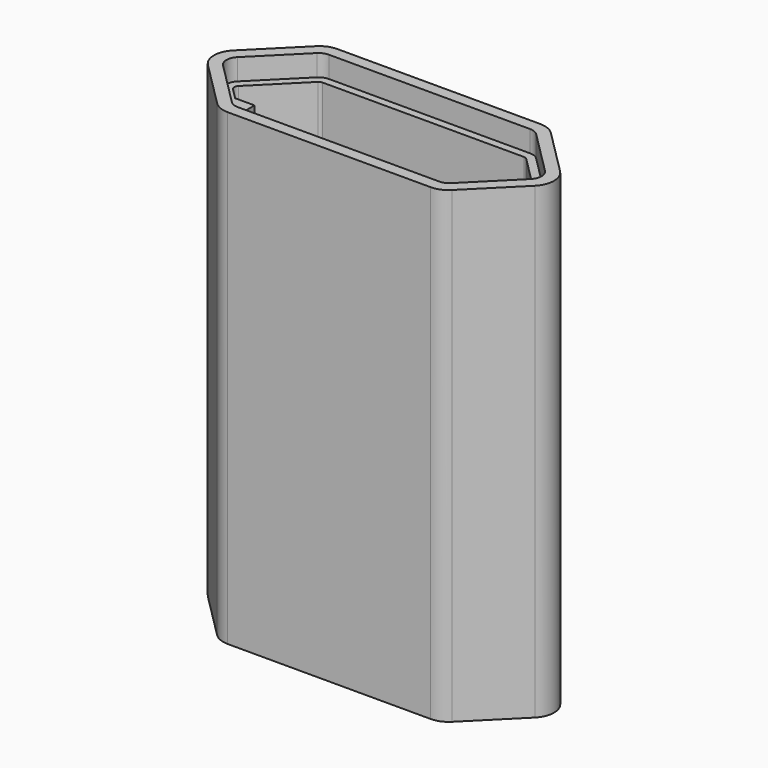
from build123d import *

# Parameters (mm, degrees)
F1_DEPTH     = 2
F2_DEPTH     = 5
F3_DEPTH     = 44
F4_DEPTH     = 46.2
F6_T1_DEPTH  = 6.8
F6_T3_DEPTH  = 13.8
F6_T9_DEPTH  = 16.371682988
F6_T15_DEPTH = 9.371682988
F6_T24_DEPTH = 9.371682988
F6_T30_DEPTH = 16.371682988
F6_T39_DEPTH = 16.371682988
F6_T45_DEPTH = 9.371682988
F6_T54_DEPTH = 16.371682988
F6_T60_DEPTH = 9.371682988


# Not quite as in the source:
# - a fillet or chamfer that OpenCascade refuses, or shapes differently, is made with other operations: its cross-section is extruded or revolved along the edge and cut away or added
# - a feature names something its author has since deleted; it is built from what else it names


with BuildPart() as f1:
    # F0 (on Top) → F1 (new body)
    with BuildSketch(Plane.XY):
        with BuildLine():
            Line((10.3671572875, 5.05), (0, 5.05))
            Line((0, 5.05), (0, 4.2))
            Line((0, 4.2), (7.7, 4.2))
            Line((7.7, 4.2), (7.7, -4.2))
            Line((7.7, -4.2), (0, -4.2))
            Line((0, -4.2), (0, -5.05))
            Line((0, -5.05), (10.3671572875, -5.05))
            ThreePointArc((10.3671572875, -5.05), (10.5584990037, -5.0119397663), (10.7207106781, -4.9035533906))
            Line((10.7207106781, -4.9035533906), (12.15, -3.4742640687))
            Line((12.15, -3.4742640687), (12.15, -1.4742640687))
            Line((12.15, -1.4742640687), (14.15, -1.4742640687))
            Line((14.15, -1.4742640687), (15.2707106781, -0.3535533906))
            ThreePointArc((15.2707106781, -0.3535533906), (15.4171572875, 0), (15.2707106781, 0.3535533906))
            Line((15.2707106781, 0.3535533906), (10.7207106781, 4.9035533906))
            ThreePointArc((10.7207106781, 4.9035533906), (10.5584990037, 5.0119397663), (10.3671572875, 5.05))
        make_face()
        Polygon((6.9, 3.4), (0, 3.4), (0, 2.8), (6.3, 2.8), (6.3, -2.8), (0, -2.8), (0, -3.4), (6.9, -3.4), align=None)
        Polygon((7.7, 4.2), (0, 4.2), (0, 3.4), (6.9, 3.4), (6.9, -3.4), (0, -3.4), (0, -4.2), (7.7, -4.2), align=None)
        with BuildLine():
            Line((10.45, 7.05), (0, 7.05))
            Line((0, 7.05), (0, 5.85))
            Line((0, 5.85), (10.3671572875, 5.85))
            ThreePointArc((10.3671572875, 5.85), (10.8646457496, 5.7510433923), (11.2863961031, 5.4692388155))
            Line((11.2863961031, 5.4692388155), (15.8363961031, 0.9192388155))
            ThreePointArc((15.8363961031, 0.9192388155), (16.2171572875, 0), (15.8363961031, -0.9192388155))
            Line((15.8363961031, -0.9192388155), (11.2863961031, -5.4692388155))
            ThreePointArc((11.2863961031, -5.4692388155), (10.8646457496, -5.7510433923), (10.3671572875, -5.85))
            Line((10.3671572875, -5.85), (0, -5.85))
            Line((0, -5.85), (0, -7.05))
            Line((0, -7.05), (10.45, -7.05))
            ThreePointArc((10.45, -7.05), (11.3301718944, -6.8749229248), (12.0763455967, -6.3763455967))
            Line((12.0763455967, -6.3763455967), (16.8263455967, -1.6263455967))
            ThreePointArc((16.8263455967, -1.6263455967), (17.5, 0), (16.8263455967, 1.6263455967))
            Line((16.8263455967, 1.6263455967), (12.0763455967, 6.3763455967))
            ThreePointArc((12.0763455967, 6.3763455967), (11.3301718944, 6.8749229248), (10.45, 7.05))
        make_face()
        with BuildLine():
            Line((10.3671572875, 5.85), (0, 5.85))
            Line((0, 5.85), (0, 5.05))
            Line((0, 5.05), (10.3671572875, 5.05))
            ThreePointArc((10.3671572875, 5.05), (10.5584990037, 5.0119397663), (10.7207106781, 4.9035533906))
            Line((10.7207106781, 4.9035533906), (15.2707106781, 0.3535533906))
            ThreePointArc((15.2707106781, 0.3535533906), (15.4171572875, 0), (15.2707106781, -0.3535533906))
            Line((15.2707106781, -0.3535533906), (14.15, -1.4742640687))
            Line((14.15, -1.4742640687), (12.15, -1.4742640687))
            Line((12.15, -1.4742640687), (12.15, -3.4742640687))
            Line((12.15, -3.4742640687), (10.7207106781, -4.9035533906))
            ThreePointArc((10.7207106781, -4.9035533906), (10.5584990037, -5.0119397663), (10.3671572875, -5.05))
            Line((10.3671572875, -5.05), (0, -5.05))
            Line((0, -5.05), (0, -5.85))
            Line((0, -5.85), (10.3671572875, -5.85))
            ThreePointArc((10.3671572875, -5.85), (10.8646457496, -5.7510433923), (11.2863961031, -5.4692388155))
            Line((11.2863961031, -5.4692388155), (15.8363961031, -0.9192388155))
            ThreePointArc((15.8363961031, -0.9192388155), (16.2171572875, 0), (15.8363961031, 0.9192388155))
            Line((15.8363961031, 0.9192388155), (11.2863961031, 5.4692388155))
            ThreePointArc((11.2863961031, 5.4692388155), (10.8646457496, 5.7510433923), (10.3671572875, 5.85))
        make_face()
    extrude(amount=-F1_DEPTH)

    # F0 (on Top) → F2 (join)
    with BuildSketch(Plane.XY):
        Polygon((7.7, 4.2), (0, 4.2), (0, 3.4), (6.9, 3.4), (6.9, -3.4), (0, -3.4), (0, -4.2), (7.7, -4.2), align=None)
    extrude(amount=F2_DEPTH)

    # F0 (on Top) → F3 (join)
    with BuildSketch(Plane.XY):
        with BuildLine():
            Line((10.3671572875, 5.85), (0, 5.85))
            Line((0, 5.85), (0, 5.05))
            Line((0, 5.05), (10.3671572875, 5.05))
            ThreePointArc((10.3671572875, 5.05), (10.5584990037, 5.0119397663), (10.7207106781, 4.9035533906))
            Line((10.7207106781, 4.9035533906), (15.2707106781, 0.3535533906))
            ThreePointArc((15.2707106781, 0.3535533906), (15.4171572875, 0), (15.2707106781, -0.3535533906))
            Line((15.2707106781, -0.3535533906), (14.15, -1.4742640687))
            Line((14.15, -1.4742640687), (12.15, -1.4742640687))
            Line((12.15, -1.4742640687), (12.15, -3.4742640687))
            Line((12.15, -3.4742640687), (10.7207106781, -4.9035533906))
            ThreePointArc((10.7207106781, -4.9035533906), (10.5584990037, -5.0119397663), (10.3671572875, -5.05))
            Line((10.3671572875, -5.05), (0, -5.05))
            Line((0, -5.05), (0, -5.85))
            Line((0, -5.85), (10.3671572875, -5.85))
            ThreePointArc((10.3671572875, -5.85), (10.8646457496, -5.7510433923), (11.2863961031, -5.4692388155))
            Line((11.2863961031, -5.4692388155), (15.8363961031, -0.9192388155))
            ThreePointArc((15.8363961031, -0.9192388155), (16.2171572875, 0), (15.8363961031, 0.9192388155))
            Line((15.8363961031, 0.9192388155), (11.2863961031, 5.4692388155))
            ThreePointArc((11.2863961031, 5.4692388155), (10.8646457496, 5.7510433923), (10.3671572875, 5.85))
        make_face()
    extrude(amount=F3_DEPTH)

    # F0 (on Top) → F4 (join)
    with BuildSketch(Plane.XY):
        with BuildLine():
            Line((10.45, 7.05), (0, 7.05))
            Line((0, 7.05), (0, 5.85))
            Line((0, 5.85), (10.3671572875, 5.85))
            ThreePointArc((10.3671572875, 5.85), (10.8646457496, 5.7510433923), (11.2863961031, 5.4692388155))
            Line((11.2863961031, 5.4692388155), (15.8363961031, 0.9192388155))
            ThreePointArc((15.8363961031, 0.9192388155), (16.2171572875, 0), (15.8363961031, -0.9192388155))
            Line((15.8363961031, -0.9192388155), (11.2863961031, -5.4692388155))
            ThreePointArc((11.2863961031, -5.4692388155), (10.8646457496, -5.7510433923), (10.3671572875, -5.85))
            Line((10.3671572875, -5.85), (0, -5.85))
            Line((0, -5.85), (0, -7.05))
            Line((0, -7.05), (10.45, -7.05))
            ThreePointArc((10.45, -7.05), (11.3301718944, -6.8749229248), (12.0763455967, -6.3763455967))
            Line((12.0763455967, -6.3763455967), (16.8263455967, -1.6263455967))
            ThreePointArc((16.8263455967, -1.6263455967), (17.5, 0), (16.8263455967, 1.6263455967))
            Line((16.8263455967, 1.6263455967), (12.0763455967, 6.3763455967))
            ThreePointArc((12.0763455967, 6.3763455967), (11.3301718944, 6.8749229248), (10.45, 7.05))
        make_face()
    extrude(amount=F4_DEPTH)

    # F5: F1 across face


with BuildPart() as f1_1:
    add(f1.part)
    add(f1.part.mirror(Plane(origin=(0, 5.8802646888, 19.9395384914), x_dir=(0, -1, 0), z_dir=(-1, 0, 0))))

    # F6: chamfer of 1 on 4 edges, made by hand

    # F6_s2 → F6_t1 (cut)
    with BuildSketch(Plane.XZ.offset(-3.4)):
        Polygon((7.9, 5), (6.9, 4), (6.9, 5), align=None)
        Polygon((-7.9, 5), (-6.9, 4), (-6.9, 5), align=None)
    extrude(amount=F6_T1_DEPTH, mode=Mode.SUBTRACT)

    # F6_s4 → F6_t3 (cut)
    with BuildSketch(Plane.YZ.offset(-6.9)):
        Polygon((4.4, 5), (3.4, 4), (3.4, 5), align=None)
        Polygon((-4.4, 5), (-3.4, 4), (-3.4, 5), align=None)
    extrude(amount=F6_T3_DEPTH, mode=Mode.SUBTRACT)


with BuildPart() as f6_tool7:
    # F6_s8 → F6_t9 (new body)
    with BuildSketch(Plane.YZ.offset(9.471682988)):
        Polygon((4.4, 5), (3.4, 4), (3.4, 5), align=None)
    extrude(amount=-F6_T9_DEPTH)

    split(bisect_by=Plane.YZ.offset(7.7), keep=Keep.BOTTOM)

    split(bisect_by=Plane.YZ.offset(6.9), keep=Keep.TOP)

    split(bisect_by=Plane.XZ.offset(-4.2), keep=Keep.TOP)


with BuildPart() as f6_tool13:
    # F6_s14 → F6_t15 (new body)
    with BuildSketch(Plane.XZ.offset(-5.971682988)):
        Polygon((7.9, 5), (6.9, 4), (6.9, 5), align=None)
    extrude(amount=F6_T15_DEPTH)

    split(bisect_by=Plane.YZ.offset(7.7), keep=Keep.BOTTOM)

    split(bisect_by=Plane.XZ.offset(-3.4), keep=Keep.BOTTOM)

    split(bisect_by=Plane.XZ.offset(-4.2), keep=Keep.TOP)


with BuildPart() as f6_tool7_1:
    add(f6_tool7.part)

    # F6_t19: intersect F6_tool13
    add(f6_tool13.part, mode=Mode.INTERSECT)


with BuildPart() as f1_2:
    add(f1_1.part)

    # F6_t5: cut F6_tool7
    add(f6_tool7_1.part, mode=Mode.SUBTRACT)


with BuildPart() as f6_tool22:
    # F6_s23 → F6_t24 (new body)
    with BuildSketch(Plane.XZ.offset(-3.4)):
        Polygon((7.9, 5), (6.9, 4), (6.9, 5), align=None)
    extrude(amount=F6_T24_DEPTH)

    split(bisect_by=Plane.YZ.offset(7.7), keep=Keep.BOTTOM)

    split(bisect_by=Plane.XZ.offset(3.4), keep=Keep.TOP)

    split(bisect_by=Plane.XZ.offset(4.2), keep=Keep.BOTTOM)


with BuildPart() as f6_tool28:
    # F6_s29 → F6_t30 (new body)
    with BuildSketch(Plane.YZ.offset(-6.9)):
        Polygon((-4.4, 5), (-3.4, 4), (-3.4, 5), align=None)
    extrude(amount=F6_T30_DEPTH)

    split(bisect_by=Plane.YZ.offset(7.7), keep=Keep.BOTTOM)

    split(bisect_by=Plane.YZ.offset(6.9), keep=Keep.TOP)

    split(bisect_by=Plane.XZ.offset(4.2), keep=Keep.BOTTOM)


with BuildPart() as f6_tool22_1:
    add(f6_tool22.part)

    # F6_t34: intersect F6_tool28
    add(f6_tool28.part, mode=Mode.INTERSECT)


with BuildPart() as f1_3:
    add(f1_2.part)

    # F6_t20: cut F6_tool22
    add(f6_tool22_1.part, mode=Mode.SUBTRACT)


with BuildPart() as f6_tool37:
    # F6_s38 → F6_t39 (new body)
    with BuildSketch(Plane.YZ.offset(6.9)):
        Polygon((4.4, 5), (3.4, 4), (3.4, 5), align=None)
    extrude(amount=-F6_T39_DEPTH)

    split(bisect_by=Plane.YZ.offset(-6.9), keep=Keep.BOTTOM)

    split(bisect_by=Plane.XZ.offset(-4.2), keep=Keep.TOP)

    split(bisect_by=Plane.YZ.offset(-7.7), keep=Keep.TOP)


with BuildPart() as f6_tool43:
    # F6_s44 → F6_t45 (new body)
    with BuildSketch(Plane.XZ.offset(-5.971682988)):
        Polygon((-7.9, 5), (-6.9, 4), (-6.9, 5), align=None)
    extrude(amount=F6_T45_DEPTH)

    split(bisect_by=Plane.XZ.offset(-3.4), keep=Keep.BOTTOM)

    split(bisect_by=Plane.XZ.offset(-4.2), keep=Keep.TOP)

    split(bisect_by=Plane.YZ.offset(-7.7), keep=Keep.TOP)


with BuildPart() as f6_tool37_1:
    add(f6_tool37.part)

    # F6_t49: intersect F6_tool43
    add(f6_tool43.part, mode=Mode.INTERSECT)


with BuildPart() as f1_4:
    add(f1_3.part)

    # F6_t35: cut F6_tool37
    add(f6_tool37_1.part, mode=Mode.SUBTRACT)


with BuildPart() as f6_tool52:
    # F6_s53 → F6_t54 (new body)
    with BuildSketch(Plane.YZ.offset(-9.471682988)):
        Polygon((-4.4, 5), (-3.4, 4), (-3.4, 5), align=None)
    extrude(amount=F6_T54_DEPTH)

    split(bisect_by=Plane.YZ.offset(-6.9), keep=Keep.BOTTOM)

    split(bisect_by=Plane.YZ.offset(-7.7), keep=Keep.TOP)

    split(bisect_by=Plane.XZ.offset(4.2), keep=Keep.BOTTOM)


with BuildPart() as f6_tool58:
    # F6_s59 → F6_t60 (new body)
    with BuildSketch(Plane.XZ.offset(-3.4)):
        Polygon((-7.9, 5), (-6.9, 4), (-6.9, 5), align=None)
    extrude(amount=F6_T60_DEPTH)

    split(bisect_by=Plane.XZ.offset(3.4), keep=Keep.TOP)

    split(bisect_by=Plane.YZ.offset(-7.7), keep=Keep.TOP)

    split(bisect_by=Plane.XZ.offset(4.2), keep=Keep.BOTTOM)


with BuildPart() as f6_tool52_1:
    add(f6_tool52.part)

    # F6_t64: intersect F6_tool58
    add(f6_tool58.part, mode=Mode.INTERSECT)


with BuildPart() as f1_5:
    add(f1_4.part)

    # F6_t50: cut F6_tool52
    add(f6_tool52_1.part, mode=Mode.SUBTRACT)


solid = f1_5.part
